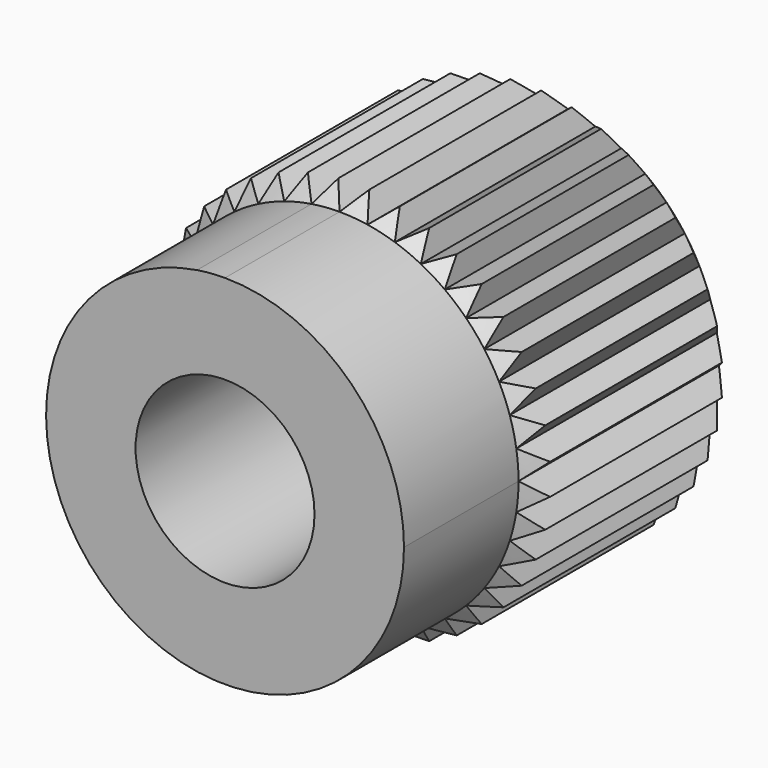
from build123d import *

# Parameters (mm, degrees)
F0_R            = 2.5
F1_DEPTH        = 11
F2_DEPTH        = 7
F2_COPIES_COUNT = 40


# Not quite as in the source:
# - a pattern or mirror of a feature is missing from the dataset's text; its kind, count and spacing are read off the source's solid


with BuildPart() as f1:
    # F0 (on Front) → F1 (new body)
    with BuildSketch(Plane.XZ):
        with BuildLine():
            ThreePointArc((-0.7821723252, 4.938441703), (-3.2472402417, -3.802029828), (5, 0))
            ThreePointArc((5, 0), (3.5355339059, 3.5355339059), (0, 5))
            ThreePointArc((0, 5), (-0.3922954786, 4.9845866687), (-0.7821723252, 4.938441703))
        make_face()
        Circle(F0_R, mode=Mode.SUBTRACT)
    extrude(amount=F1_DEPTH)

    # F0 (on Front) → F2 (join)
    with BuildSketch(Plane.XZ):
        with BuildLine():
            ThreePointArc((-0.7821723252, 4.938441703), (-0.3922954786, 4.9845866687), (0, 5))
            Line((0, 5), (-0.4315250265, 5.4830453355))
            Line((-0.4315250265, 5.4830453355), (-0.7821723252, 4.938441703))
        make_face()
    f2 = extrude(amount=F2_DEPTH)

    # F2_copies: F2 ×40 about axis
    f2_copies_axis = Axis((0, 0, 0), (0, 1, 0))
    for i in range(1, F2_COPIES_COUNT):
        add(f2.rotate(f2_copies_axis, i * 360 / F2_COPIES_COUNT))

    # F3 (on Top) → F4 (revolve, cut)
    with BuildSketch(Plane.XY):
        Polygon((8, 0), (5, 0), (7, -2), (7, -5), (5, -7), (8, -7), align=None)
    revolve(axis=Axis((0, -7.7233230695, 0), (0, -1, 0)), mode=Mode.SUBTRACT)


solid = f1.part
